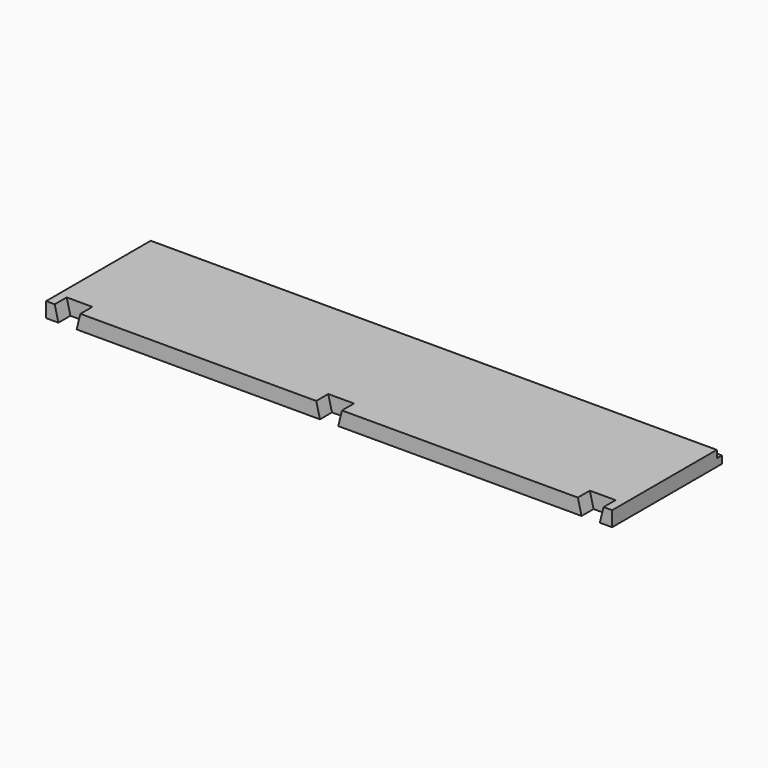
from build123d import *

# Parameters (mm, degrees)
F0_W     = 838.2
F0_H     = 203.2
F1_DEPTH = 22.225
F2_W     = 838.2
F2_H     = 9.525
F3_DEPTH = 11.1125
F5_DEPTH = 22.225


# Not quite as in the source:
# - a feature names something its author has since deleted; it is built from what else it names


with BuildPart() as f1:
    # F0 (on Top) → F1 (new body)
    with BuildSketch(Plane.XY):
        with Locations((419.1, -101.6)):
            Rectangle(F0_W, F0_H)
    extrude(amount=F1_DEPTH)

    # F2 (on face) → F3 (cut)
    with BuildSketch(Plane.XY.offset(22.225)):
        with Locations((419.1, -4.7625)):
            Rectangle(F2_W, F2_H)
    extrude(amount=-F3_DEPTH, mode=Mode.SUBTRACT)

    # F4 (on face) → F5 (cut)
    with BuildSketch(Plane.XZ.offset(203.2)):
        Polygon((438.15, 22.225), (400.05, 22.225), (405.5913148632, 0), (432.6086851368, 0), align=None)
        Polygon((45.2586851368, 0), (50.8, 22.225), (12.7, 22.225), (18.2413148632, 0), align=None)
        Polygon((825.5, 22.225), (787.4, 22.225), (792.9413148632, 0), (819.9586851368, 0), align=None)
    extrude(amount=-F5_DEPTH, mode=Mode.SUBTRACT)


solid = f1.part
